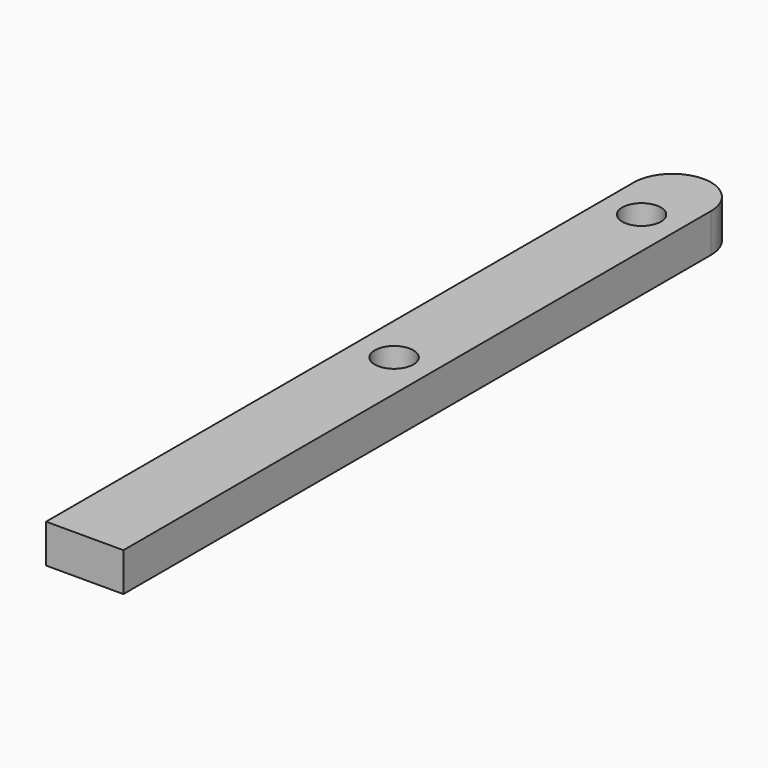
from build123d import *

# Parameters (mm, degrees)
F0_R     = 2.5
F1_DEPTH = 5
F2_R     = 4.99999


# Not quite as in the source:
# - a fillet or chamfer is up to 0.001 mm smaller than in the source, because OpenCascade refuses the exact size


with BuildPart() as f1:
    # F0 (on Top) → F1 (new body)
    with BuildSketch(Plane.XY):
        Polygon((0, 50), (0, 0), (10, 0), (10, 100), (0, 100), align=None)
        with Locations((5, 50)):
            Circle(F0_R, mode=Mode.SUBTRACT)
        with Locations((5, 90)):
            Circle(F0_R, mode=Mode.SUBTRACT)
    extrude(amount=F1_DEPTH)

    # F2 (radius 5 in the source; OpenCascade refuses exactly that, so slightly less here)
    f2_edges = [f1.edges().sort_by_distance(p)[0] for p in [
        (0, 100, 2.5),
        (10, 100, 2.5),
    ]]
    fillet(f2_edges, radius=F2_R)


solid = f1.part
